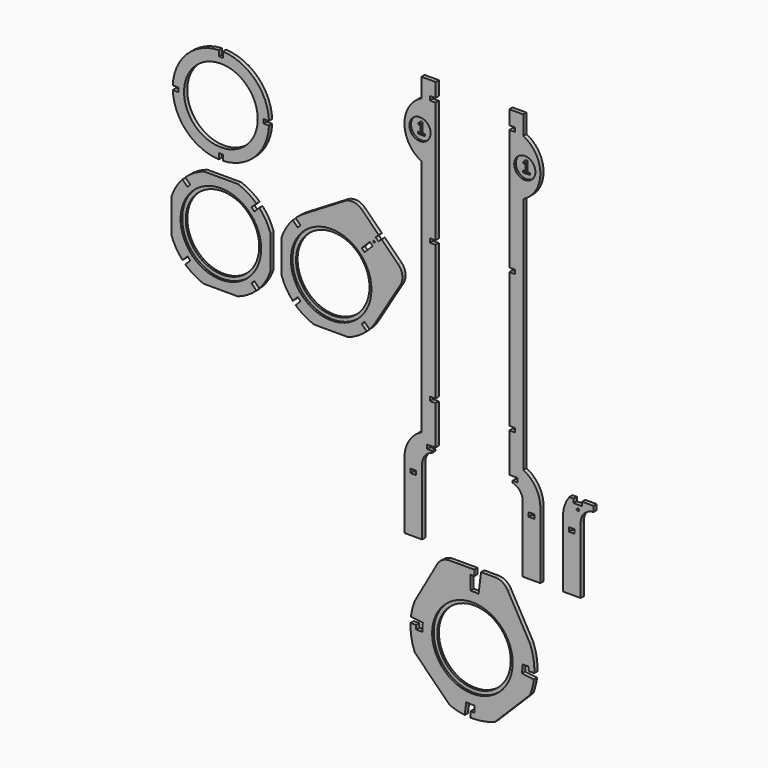
from build123d import *

# Parameters (mm, degrees)
F1_R     = 165.5919642374
F2_DEPTH = 18.034
F1_R_2   = 180.975
F1_R_3   = 3.81
F1_W     = 25.4
F1_H     = 18.034
F1_R_4   = 47.625
F1_W_2   = 18.034
F1_H_2   = 25.4
F1_R_5   = 5.334
F1_R_6   = 165.1
F3_DEPTH = 9.017


# Not quite as in the source:
# - a variable given as a bare number and used for a length is read in inches; the dataset says mm whatever the document's units were
# - a feature names something its author has since deleted; it is built from what else it names


with BuildPart() as f2:
    # F1 (on Front) → F2 (new body)
    with BuildSketch(Plane.XZ):
        with BuildLine():
            Line((190.9919642374, 517.017), (216.2040145269, 517.017))
            ThreePointArc((216.2040145269, 517.017), (153.0122253066, 661.0122253066), (9.017, 724.2040145269))
            Line((9.017, 724.2040145269), (9.017, 698.9919642374))
            Line((9.017, 698.9919642374), (-9.017, 698.9919642374))
            Line((-9.017, 698.9919642374), (-9.017, 724.2040145269))
            ThreePointArc((-9.017, 724.2040145269), (-153.0122253066, 661.0122253066), (-216.2040145269, 517.017))
            Line((-216.2040145269, 517.017), (-190.9919642374, 517.017))
            Line((-190.9919642374, 517.017), (-190.9919642374, 498.983))
            Line((-190.9919642374, 498.983), (-216.2040145269, 498.983))
            ThreePointArc((-216.2040145269, 498.983), (-153.0122253066, 354.9877746934), (-9.017, 291.7959854731))
            Line((-9.017, 291.7959854731), (-9.017, 317.0080357626))
            Line((-9.017, 317.0080357626), (9.017, 317.0080357626))
            Line((9.017, 317.0080357626), (9.017, 291.7959854731))
            ThreePointArc((9.017, 291.7959854731), (153.0122253066, 354.9877746934), (216.2040145269, 498.983))
            Line((216.2040145269, 498.983), (190.9919642374, 498.983))
            Line((190.9919642374, 498.983), (190.9919642374, 517.017))
        make_face()
        with Locations((0, 508)):
            Circle(F1_R, mode=Mode.SUBTRACT)
    extrude(amount=F2_DEPTH)


with BuildPart() as f2b:
    # F1 (on Front) → F2, piece 2 (new body)
    with BuildSketch(Plane.XZ):
        with BuildLine():
            Line((76.2, 222.25), (-76.2, 222.25))
            ThreePointArc((-76.2, 222.25), (-120.5248687802, 201.6810811789), (-159.6363613864, 172.3883250783))
            Line((-159.6363613864, 172.3883250783), (-137.3081160911, 150.0600797831))
            Line((-137.3081160911, 150.0600797831), (-150.0600797831, 137.3081160911))
            Line((-150.0600797831, 137.3081160911), (-172.3883250783, 159.6363613864))
            ThreePointArc((-172.3883250783, 159.6363613864), (-201.6810811789, 120.5248687802), (-222.25, 76.2))
            Line((-222.25, 76.2), (-222.25, -76.2))
            ThreePointArc((-222.25, -76.2), (-201.6810811789, -120.5248687802), (-172.3883250783, -159.6363613864))
            Line((-172.3883250783, -159.6363613864), (-150.0600797831, -137.3081160911))
            Line((-150.0600797831, -137.3081160911), (-137.3081160911, -150.0600797831))
            Line((-137.3081160911, -150.0600797831), (-159.6363613864, -172.3883250783))
            ThreePointArc((-159.6363613864, -172.3883250783), (-120.5248687802, -201.6810811789), (-76.2, -222.25))
            Line((-76.2, -222.25), (76.2, -222.25))
            ThreePointArc((76.2, -222.25), (120.5248687802, -201.6810811789), (159.6363613864, -172.3883250783))
            Line((159.6363613864, -172.3883250783), (137.3081160911, -150.0600797831))
            Line((137.3081160911, -150.0600797831), (150.0600797831, -137.3081160911))
            Line((150.0600797831, -137.3081160911), (172.3883250783, -159.6363613864))
            ThreePointArc((172.3883250783, -159.6363613864), (201.6810811789, -120.5248687802), (222.25, -76.2))
            Line((222.25, -76.2), (222.25, 76.2))
            ThreePointArc((222.25, 76.2), (201.6810811789, 120.5248687802), (172.3883250783, 159.6363613864))
            Line((172.3883250783, 159.6363613864), (150.0600797831, 137.3081160911))
            Line((150.0600797831, 137.3081160911), (137.3081160911, 150.0600797831))
            Line((137.3081160911, 150.0600797831), (159.6363613864, 172.3883250783))
            ThreePointArc((159.6363613864, 172.3883250783), (120.5248687802, 201.6810811789), (76.2, 222.25))
        make_face()
        Circle(F1_R_2, mode=Mode.SUBTRACT)
    extrude(amount=F2_DEPTH)

    # F1 (on Front) → F3 (join)
    with BuildSketch(Plane.XZ):
        Circle(F1_R_2)
        Circle(F1_R_6, mode=Mode.SUBTRACT)
    extrude(amount=F3_DEPTH)


with BuildPart() as f2c:
    # F1 (on Front) → F2, piece 3 (new body)
    with BuildSketch(Plane.XZ):
        with BuildLine():
            Line((632.6081160911, -150.0600797831), (645.3600797831, -137.3081160911))
            Line((645.3600797831, -137.3081160911), (667.6883250783, -159.6363613864))
            ThreePointArc((667.6883250783, -159.6363613864), (682.3835034472, -142.1311550573), (695.3082811454, -123.2809392131))
            Line((695.3082811454, -123.2809392131), (697.5672203454, -119.5385882205))
            ThreePointArc((697.5672203454, -119.5385882205), (708.6618426516, -98.3779782285), (717.55, -76.2))
            Line((717.55, -76.2), (717.55, 76.2))
            ThreePointArc((717.55, 76.2), (696.9810811789, 120.5248687802), (667.6883250783, 159.6363613864))
            Line((667.6883250783, 159.6363613864), (645.3600797831, 137.3081160911))
            Line((645.3600797831, 137.3081160911), (632.6081160911, 150.0600797831))
            Line((632.6081160911, 150.0600797831), (654.9363613864, 172.3883250783))
            ThreePointArc((654.9363613864, 172.3883250783), (615.8248687802, 201.6810811789), (571.5, 222.25))
            Line((571.5, 222.25), (419.1, 222.25))
            ThreePointArc((419.1, 222.25), (396.9220217715, 213.3618426516), (375.7614117795, 202.2672203454))
            Line((375.7614117795, 202.2672203454), (372.0190607869, 200.0082811454))
            ThreePointArc((372.0190607869, 200.0082811454), (353.1688449427, 187.0835034472), (335.6636386136, 172.3883250783))
            Line((335.6636386136, 172.3883250783), (357.9918839089, 150.0600797831))
            Line((357.9918839089, 150.0600797831), (345.2399202169, 137.3081160911))
            Line((345.2399202169, 137.3081160911), (322.9116749217, 159.6363613864))
            ThreePointArc((322.9116749217, 159.6363613864), (293.6189188211, 120.5248687802), (273.05, 76.2))
            Line((273.05, 76.2), (273.05, -76.2))
            ThreePointArc((273.05, -76.2), (293.6189188211, -120.5248687802), (322.9116749217, -159.6363613864))
            Line((322.9116749217, -159.6363613864), (345.2399202169, -137.3081160911))
            Line((345.2399202169, -137.3081160911), (357.9918839089, -150.0600797831))
            Line((357.9918839089, -150.0600797831), (335.6636386136, -172.3883250783))
            ThreePointArc((335.6636386136, -172.3883250783), (374.7751312198, -201.6810811789), (419.1, -222.25))
            Line((419.1, -222.25), (571.5, -222.25))
            ThreePointArc((571.5, -222.25), (615.8248687802, -201.6810811789), (654.9363613864, -172.3883250783))
            Line((654.9363613864, -172.3883250783), (632.6081160911, -150.0600797831))
        make_face()
        with Locations((495.3, 0)):
            Circle(F1_R_2, mode=Mode.SUBTRACT)
        with BuildLine():
            ThreePointArc((571.5, 222.25), (615.8248687802, 201.6810811789), (654.9363613864, 172.3883250783))
            Line((654.9363613864, 172.3883250783), (668.5291405754, 185.9811042673))
            Line((668.5291405754, 185.9811042673), (695.4699089386, 212.9218726305))
            Line((695.4699089386, 212.9218726305), (708.9402931202, 226.3922568122))
            Line((708.9402931202, 226.3922568122), (633.7268071321, 301.6057428003))
            ThreePointArc((633.7268071321, 301.6057428003), (596.5005285207, 319.738931689), (556.0106569847, 311.0683687593))
            Line((556.0106569847, 311.0683687593), (375.7614117795, 202.2672203454))
            ThreePointArc((375.7614117795, 202.2672203454), (396.9220217715, 213.3618426516), (419.1, 222.25))
            Line((419.1, 222.25), (571.5, 222.25))
        make_face()
        with BuildLine():
            ThreePointArc((717.55, -76.2), (708.6618426516, -98.3779782285), (697.5672203454, -119.5385882205))
            Line((697.5672203454, -119.5385882205), (806.3683687593, 60.7106569847))
            ThreePointArc((806.3683687593, 60.7106569847), (815.038931689, 101.2005285207), (796.9057428003, 138.4268071321))
            Line((796.9057428003, 138.4268071321), (721.6922568122, 213.6402931202))
            Line((721.6922568122, 213.6402931202), (708.2218726305, 200.1699089386))
            Line((708.2218726305, 200.1699089386), (681.2811042673, 173.2291405754))
            Line((681.2811042673, 173.2291405754), (667.6883250783, 159.6363613864))
            ThreePointArc((667.6883250783, 159.6363613864), (696.9810811789, 120.5248687802), (717.55, 76.2))
            Line((717.55, 76.2), (717.55, -76.2))
        make_face()
        Polygon((668.5291405754, 185.9811042673), (681.2811042673, 173.2291405754), (708.2218726305, 200.1699089386), (695.4699089386, 212.9218726305), align=None)
        with Locations((688.375506603, 193.075506603)):
            Circle(F1_R_3, mode=Mode.SUBTRACT)
    extrude(amount=F2_DEPTH)

    # F1 (on Front) → F3, piece 2 (join)
    with BuildSketch(Plane.XZ):
        with Locations((495.3, 0)):
            Circle(F1_R_2)
        with Locations((495.3, 0)):
            Circle(F1_R_6, mode=Mode.SUBTRACT)
    extrude(amount=F3_DEPTH)


with BuildPart() as f2d:
    # F1 (on Front) → F2, piece 4 (new body)
    with BuildSketch(Plane.XZ):
        with BuildLine():
            Line((1358.9, 914.4), (1295.4, 914.4))
            Line((1295.4, 914.4), (1295.4, 850.9))
            Line((1295.4, 850.9), (1320.8, 850.9))
            Line((1320.8, 850.9), (1320.8, 832.866))
            Line((1320.8, 832.866), (1295.4, 832.866))
            Line((1295.4, 832.866), (1295.4, 288.417))
            Line((1295.4, 288.417), (1320.8, 288.417))
            Line((1320.8, 288.417), (1320.8, 270.383))
            Line((1320.8, 270.383), (1295.4, 270.383))
            Line((1295.4, 270.383), (1295.4, -337.566))
            Line((1295.4, -337.566), (1320.8, -337.566))
            Line((1320.8, -337.566), (1320.8, -355.6))
            Line((1320.8, -355.6), (1295.4, -355.6))
            Line((1295.4, -355.6), (1295.4, -531.241))
            Line((1295.4, -531.241), (1333.0080357626, -531.241))
            Line((1333.0080357626, -531.241), (1333.0080357626, -549.275))
            Line((1333.0080357626, -549.275), (1310.7830357626, -549.275))
            Line((1310.7830357626, -549.275), (1310.7830357626, -557.6193233733))
            ThreePointArc((1310.7830357626, -557.6193233733), (1343.1864377066, -579.132042475), (1355.725, -615.95))
            Line((1355.725, -615.95), (1355.725, -914.4))
            Line((1355.725, -914.4), (1435.1, -914.4))
            Line((1435.1, -914.4), (1435.1, -615.95))
            ThreePointArc((1435.1, -615.95), (1414.5365602995, -542.994054389), (1358.9, -491.5159210666))
            Line((1358.9, -491.5159210666), (1358.9, 580.4159210666))
            ThreePointArc((1358.9, 580.4159210666), (1435.1, 704.85), (1358.9, 829.2840789334))
            Line((1358.9, 829.2840789334), (1358.9, 914.4))
        make_face()
        with Locations((1395.4125, -659.892)):
            Rectangle(F1_W, F1_H, mode=Mode.SUBTRACT)
        with Locations((1365.25, 704.85)):
            Circle(F1_R_4, mode=Mode.SUBTRACT)
    extrude(amount=F2_DEPTH)

    # F1 (on Front) → F3, piece 3 (join)
    with BuildSketch(Plane.XZ):
        with Locations((1365.25, 704.85)):
            Circle(F1_R_4)
        Polygon((1361.1225, 731.2025), (1369.3775, 731.2025), (1369.3775, 686.7525), (1381.125, 686.7525), (1381.125, 678.4975), (1349.375, 678.4975), (1349.375, 686.7525), (1361.1225, 686.7525), (1361.1225, 719.3693540915), (1355.2894696578, 713.3786742806), (1349.375, 719.1375), align=None, mode=Mode.SUBTRACT)
    extrude(amount=F3_DEPTH)


with BuildPart() as f2e:
    # F1 (on Front) → F2, piece 5 (new body)
    with BuildSketch(Plane.XZ):
        with BuildLine():
            Line((938.8160715252, 850.9), (964.2160715252, 850.9))
            Line((964.2160715252, 850.9), (964.2160715252, 914.4))
            Line((964.2160715252, 914.4), (900.7160715252, 914.4))
            Line((900.7160715252, 914.4), (900.7160715252, 829.2840789334))
            ThreePointArc((900.7160715252, 829.2840789334), (824.5160715252, 704.85), (900.7160715252, 580.4159210666))
            Line((900.7160715252, 580.4159210666), (900.7160715252, -491.5159210666))
            ThreePointArc((900.7160715252, -491.5159210666), (845.0795112256, -542.994054389), (824.5160715252, -615.95))
            Line((824.5160715252, -615.95), (824.5160715252, -914.4))
            Line((824.5160715252, -914.4), (903.8910715252, -914.4))
            Line((903.8910715252, -914.4), (903.8910715252, -615.95))
            ThreePointArc((903.8910715252, -615.95), (916.4296338185, -579.132042475), (948.8330357626, -557.6193233733))
            Line((948.8330357626, -557.6193233733), (948.8330357626, -549.275))
            Line((948.8330357626, -549.275), (926.6080357626, -549.275))
            Line((926.6080357626, -549.275), (926.6080357626, -531.241))
            Line((926.6080357626, -531.241), (964.2160715252, -531.241))
            Line((964.2160715252, -531.241), (964.2160715252, -355.6))
            Line((964.2160715252, -355.6), (938.8160715252, -355.6))
            Line((938.8160715252, -355.6), (938.8160715252, -337.566))
            Line((938.8160715252, -337.566), (964.2160715252, -337.566))
            Line((964.2160715252, -337.566), (964.2160715252, 270.383))
            Line((964.2160715252, 270.383), (938.8160715252, 270.383))
            Line((938.8160715252, 270.383), (938.8160715252, 288.417))
            Line((938.8160715252, 288.417), (964.2160715252, 288.417))
            Line((964.2160715252, 288.417), (964.2160715252, 832.866))
            Line((964.2160715252, 832.866), (938.8160715252, 832.866))
            Line((938.8160715252, 832.866), (938.8160715252, 850.9))
        make_face()
        with Locations((864.2035715252, -659.892)):
            Rectangle(F1_W, F1_H, mode=Mode.SUBTRACT)
        with Locations((894.3660715252, 704.85)):
            Circle(F1_R_4, mode=Mode.SUBTRACT)
    extrude(amount=F2_DEPTH)

    # F1 (on Front) → F3, piece 4 (join)
    with BuildSketch(Plane.XZ):
        with Locations((894.3660715252, 704.85)):
            Circle(F1_R_4)
        Polygon((890.2385715252, 731.2025), (898.4935715252, 731.2025), (898.4935715252, 686.7525), (910.2410715252, 686.7525), (910.2410715252, 678.4975), (878.4910715252, 678.4975), (878.4910715252, 686.7525), (890.2385715252, 686.7525), (890.2385715252, 719.3693540915), (884.405541183, 713.3786742806), (878.4910715252, 719.1375), align=None, mode=Mode.SUBTRACT)
    extrude(amount=F3_DEPTH)


with BuildPart() as f2f:
    # F1 (on Front) → F2, piece 6 (new body)
    with BuildSketch(Plane.XZ):
        with BuildLine():
            Line((1138.8250357626, -1522.7583515293), (1138.8250357626, -1548.1583515293))
            ThreePointArc((1138.8250357626, -1548.1583515293), (1185.9317567407, -1542.5866885195), (1231.4080357626, -1529.0961497485))
            Line((1231.4080357626, -1529.0961497485), (1388.904185511, -1371.6))
            ThreePointArc((1388.904185511, -1371.6), (1399.5496367324, -1338.504332131), (1405.9858087557, -1304.339663933))
            Line((1405.9858087557, -1304.339663933), (1352.432962756, -1297.6809574254))
            ThreePointArc((1352.432962756, -1297.6809574254), (1353.3943076174, -1288.3649819182), (1353.9659872918, -1279.017))
            Line((1353.9659872918, -1279.017), (1353.9659872918, -1260.983))
            Line((1353.9659872918, -1260.983), (1382.5663872918, -1260.983))
            Line((1382.5663872918, -1260.983), (1407.9663872918, -1260.983))
            ThreePointArc((1407.9663872918, -1260.983), (1402.3947242821, -1213.8762790219), (1388.904185511, -1168.4))
            Line((1388.904185511, -1168.4), (1350.4390125581, -1100.3670229799))
            ThreePointArc((1350.4390125581, -1100.3670229799), (1267.9762495298, -1028.4158127715), (1164.1476996956, -993.8222270069))
            Line((1164.1476996956, -993.8222270069), (1157.4889931879, -1047.3750730066))
            ThreePointArc((1157.4889931879, -1047.3750730066), (1148.1730176808, -1046.4137281452), (1138.8250357626, -1045.8420484707))
            Line((1138.8250357626, -1045.8420484707), (1120.7910357626, -1045.8420484707))
            Line((1120.7910357626, -1045.8420484707), (1120.7910357626, -1017.2416484707))
            Line((1120.7910357626, -1017.2416484707), (1120.7910357626, -991.8416484707))
            ThreePointArc((1120.7910357626, -991.8416484707), (1002.808084819, -1022.3623871969), (909.177058967, -1100.3670229799))
            Line((909.177058967, -1100.3670229799), (870.7118860141, -1168.4))
            ThreePointArc((870.7118860141, -1168.4), (860.0664347928, -1201.495667869), (853.6302627694, -1235.660336067))
            Line((853.6302627694, -1235.660336067), (907.1831087692, -1242.3190425746))
            ThreePointArc((907.1831087692, -1242.3190425746), (906.2217639078, -1251.6350180818), (905.6500842333, -1260.983))
            Line((905.6500842333, -1260.983), (905.6500842333, -1279.017))
            Line((905.6500842333, -1279.017), (877.0496842333, -1279.017))
            Line((877.0496842333, -1279.017), (851.6496842333, -1279.017))
            ThreePointArc((851.6496842333, -1279.017), (857.221347243, -1326.1237209781), (870.7118860141, -1371.6))
            Line((870.7118860141, -1371.6), (1028.2080357626, -1529.0961497485))
            ThreePointArc((1028.2080357626, -1529.0961497485), (1061.3037036315, -1539.7416009698), (1095.4683718296, -1546.1777729931))
            Line((1095.4683718296, -1546.1777729931), (1102.1270783372, -1492.6249269934))
            ThreePointArc((1102.1270783372, -1492.6249269934), (1111.4430538444, -1493.5862718548), (1120.7910357626, -1494.1579515293))
            Line((1120.7910357626, -1494.1579515293), (1138.8250357626, -1494.1579515293))
            Line((1138.8250357626, -1494.1579515293), (1138.8250357626, -1522.7583515293))
        make_face()
        with Locations((1129.8080357626, -1270)):
            Circle(F1_R_2, mode=Mode.SUBTRACT)
        with Locations((864.3496842333, -1270)):
            Rectangle(F1_W, F1_H)
        with Locations((1395.2663872918, -1270)):
            Rectangle(F1_W, F1_H)
        with Locations((1129.8080357626, -1535.4583515293)):
            Rectangle(F1_W_2, F1_H_2)
        with BuildLine():
            Line((971.8758280132, -989.4723204152), (909.177058967, -1100.3670229799))
            ThreePointArc((909.177058967, -1100.3670229799), (1002.808084819, -1022.3623871969), (1120.7910357626, -991.8416484707))
            Line((1120.7910357626, -991.8416484707), (1120.7910357626, -982.625192023))
            Line((1120.7910357626, -982.625192023), (1120.7910357626, -957.225192023))
            Line((1120.7910357626, -957.225192023), (1027.1524778417, -957.225192023))
            ThreePointArc((1027.1524778417, -957.225192023), (995.154879081, -965.8762752283), (971.8758280132, -989.4723204152))
        make_face()
        with Locations((1129.8080357626, -969.925192023)):
            Rectangle(F1_W_2, F1_H_2)
        with BuildLine():
            ThreePointArc((1164.1476996956, -993.8222270069), (1267.9762495298, -1028.4158127715), (1350.4390125581, -1100.3670229799))
            Line((1350.4390125581, -1100.3670229799), (1287.7402435119, -989.4723204152))
            ThreePointArc((1287.7402435119, -989.4723204152), (1264.4611924441, -965.8762752283), (1232.4635936834, -957.225192023))
            Line((1232.4635936834, -957.225192023), (1168.6981378741, -957.225192023))
            Line((1168.6981378741, -957.225192023), (1164.1476996956, -993.8222270069))
        make_face()
    extrude(amount=F2_DEPTH)

    # F1 (on Front) → F3, piece 5 (join)
    with BuildSketch(Plane.XZ):
        with Locations((1129.8080357626, -1270)):
            Circle(F1_R_2)
        with Locations((1129.8080357626, -1270)):
            Circle(F1_R_6, mode=Mode.SUBTRACT)
    extrude(amount=F3_DEPTH)


with BuildPart() as f2g:
    # F1 (on Front) → F2, piece 7 (new body)
    with BuildSketch(Plane.XZ):
        with BuildLine():
            Line((1616.075, -914.4), (1616.075, -615.95))
            ThreePointArc((1616.075, -615.95), (1632.6485034754, -574.4179379653), (1673.262307977, -555.706655855))
            Line((1673.262307977, -555.706655855), (1673.262307977, -531.241))
            Line((1673.262307977, -531.241), (1622.462307977, -531.241))
            Line((1622.462307977, -531.241), (1622.462307977, -549.275))
            Line((1622.462307977, -549.275), (1584.362307977, -549.275))
            Line((1584.362307977, -549.275), (1584.362307977, -531.241))
            Line((1584.362307977, -531.241), (1565.312307977, -531.241))
            ThreePointArc((1565.312307977, -531.241), (1544.0462305493, -571.2446344138), (1536.7, -615.95))
            Line((1536.7, -615.95), (1536.7, -914.4))
            Line((1536.7, -914.4), (1616.075, -914.4))
        make_face()
        with Locations((1576.3875, -659.892)):
            Rectangle(F1_W, F1_H, mode=Mode.SUBTRACT)
        with Locations((1603.412307977, -569.341)):
            Circle(F1_R_5, mode=Mode.SUBTRACT)
    extrude(amount=F2_DEPTH)


solid = Compound([f2.part, f2b.part, f2c.part, f2d.part, f2e.part, f2f.part, f2g.part])
